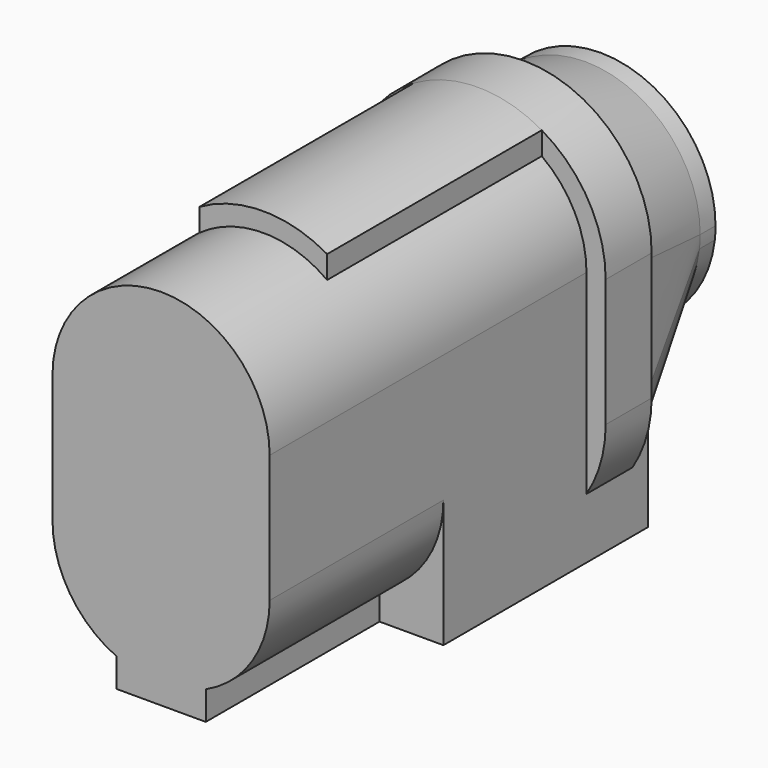
from build123d import *

# Parameters (mm, degrees)
F1_DEPTH  = 78.74
F4_W      = 50.8
F4_H      = 25.4
F6_DEPTH  = 11.43
F7_W      = 48.6228571429
F7_H      = 23.7671428571
F10_DEPTH = 3.81
F12_DEPTH = 53.34
F14_DEPTH = 38.1
F16_D     = 6.7564
F16_DEPTH = 7.62
F16_TIP   = 2.0298273432


with BuildPart() as f1:
    # F0 (on Front) → F1 (new body)
    with BuildSketch(Plane.XZ):
        with BuildLine():
            Line((-21.59, 12.7), (-21.59, -12.7))
            ThreePointArc((-21.59, -12.7), (0, -34.29), (21.59, -12.7))
            Line((21.59, -12.7), (21.59, 0))
            Line((21.59, 0), (21.59, 12.7))
            ThreePointArc((21.59, 12.7), (0, 34.29), (-21.59, 12.7))
        make_face()
    extrude(amount=F1_DEPTH)

    # F4 (on Front) → F5 section 0
    with BuildSketch(Plane.XZ):
        with BuildLine():
            Line((-25.4, 12.7), (25.4, 12.7))
            ThreePointArc((25.4, 12.7), (0, 38.1), (-25.4, 12.7))
        make_face()
    # F3 (on offset) → F5 section 1
    with BuildSketch(Plane.XZ.offset(-26.67)):
        with BuildLine():
            Line((-22.86, 8.89), (22.86, 8.89))
            ThreePointArc((22.86, 8.89), (0, 31.75), (-22.86, 8.89))
        make_face()
    loft()

    # F4 (on Front) → F6 (join)
    with BuildSketch(Plane.XZ):
        with BuildLine():
            Line((-25.4, 12.7), (25.4, 12.7))
            ThreePointArc((25.4, 12.7), (0, 38.1), (-25.4, 12.7))
        make_face()
        Rectangle(F4_W, F4_H)
        with BuildLine():
            ThreePointArc((-25.4, -12.7), (0, -38.1), (25.4, -12.7))
            Line((25.4, -12.7), (-25.4, -12.7))
        make_face()
    extrude(amount=-F6_DEPTH)

    # F7 (on face) → F8 section 0
    with BuildSketch(Plane(origin=(0, 11.43, 0), x_dir=(-1, 0, 0), z_dir=(0, 1, 0))):
        with Locations((0, -0.8164285714)):
            Rectangle(F7_W, F7_H)
    # F3 (on offset) → F8 section 1
    with BuildSketch(Plane.XZ.offset(-26.67)):
        with BuildLine():
            ThreePointArc((22.7188888889, 6.3539227823), (22.8246949596, 7.62), (22.86, 8.89))
            Line((22.86, 8.89), (-22.86, 8.89))
            ThreePointArc((-22.86, 8.89), (-22.8245852305, 7.61802946), (-22.7184506514, 6.35))
            Line((-22.7184506514, 6.35), (22.7188888889, 6.3539227823))
        make_face()
    loft()

    # F3 (on offset) → F9 section 0
    with BuildSketch(Plane.XZ.offset(-26.67)):
        with BuildLine():
            ThreePointArc((-22.7184506514, 6.35), (0.0019735927, -13.9699999148), (22.7188888889, 6.3539227823))
            Line((22.7188888889, 6.3539227823), (-22.7184506514, 6.35))
        make_face()
    # F7 (on face) → F9 section 1
    with BuildSketch(Plane(origin=(0, 11.43, 0), x_dir=(-1, 0, 0), z_dir=(0, 1, 0))):
        with BuildLine():
            Line((24.3114285714, -12.7), (-24.3114285714, -12.7))
            ThreePointArc((-24.3114285714, -12.7), (0, -37.0114285714), (24.3114285714, -12.7))
        make_face()
    loft()

    # F3 (on offset) → F10 (join)
    with BuildSketch(Plane.XZ.offset(-26.67)):
        with BuildLine():
            Line((-22.86, 8.89), (22.86, 8.89))
            ThreePointArc((22.86, 8.89), (0, 31.75), (-22.86, 8.89))
        make_face()
        with BuildLine():
            ThreePointArc((22.7188888889, 6.3539227823), (22.8246949596, 7.62), (22.86, 8.89))
            Line((22.86, 8.89), (-22.86, 8.89))
            ThreePointArc((-22.86, 8.89), (-22.8245852305, 7.61802946), (-22.7184506514, 6.35))
            Line((-22.7184506514, 6.35), (22.7188888889, 6.3539227823))
        make_face()
        with BuildLine():
            ThreePointArc((-22.7184506514, 6.35), (0.0019735927, -13.9699999148), (22.7188888889, 6.3539227823))
            Line((22.7188888889, 6.3539227823), (-22.7184506514, 6.35))
        make_face()
    extrude(amount=-F10_DEPTH)

    # F11 (on Front) → F12 (join)
    with BuildSketch(Plane.XZ):
        with BuildLine():
            Line((12.7, 12.7), (12.7, 34.6970452561))
            ThreePointArc((12.7, 34.6970452561), (0, 38.1), (-12.7, 34.6970452561))
            Line((-12.7, 34.6970452561), (-12.7, 12.7))
            Line((-12.7, 12.7), (12.7, 12.7))
        make_face()
    extrude(amount=F12_DEPTH)

    # F13 (on Top) → F14 (join)
    with BuildSketch(Plane.XY):
        Polygon((21.59, -35.56), (21.59, 15.24), (-21.59, 15.24), (-21.59, -35.56), (-8.89, -35.56), (-8.89, -78.74), (8.89, -78.74), (8.89, -35.56), align=None)
    extrude(amount=-F14_DEPTH)

    # F16
    with Locations(Plane(origin=(0, 0, -38.1), x_dir=(1, 0, 0), z_dir=(0, 0, -1))):
        with Locations((0, 55.88)):
            Hole(F16_D / 2, depth=F16_DEPTH)
            with Locations((0, 0, -(F16_DEPTH + F16_TIP / 2))):  # 118° drill point
                Cone(0, F16_D / 2, F16_TIP, mode=Mode.SUBTRACT)


solid = f1.part
